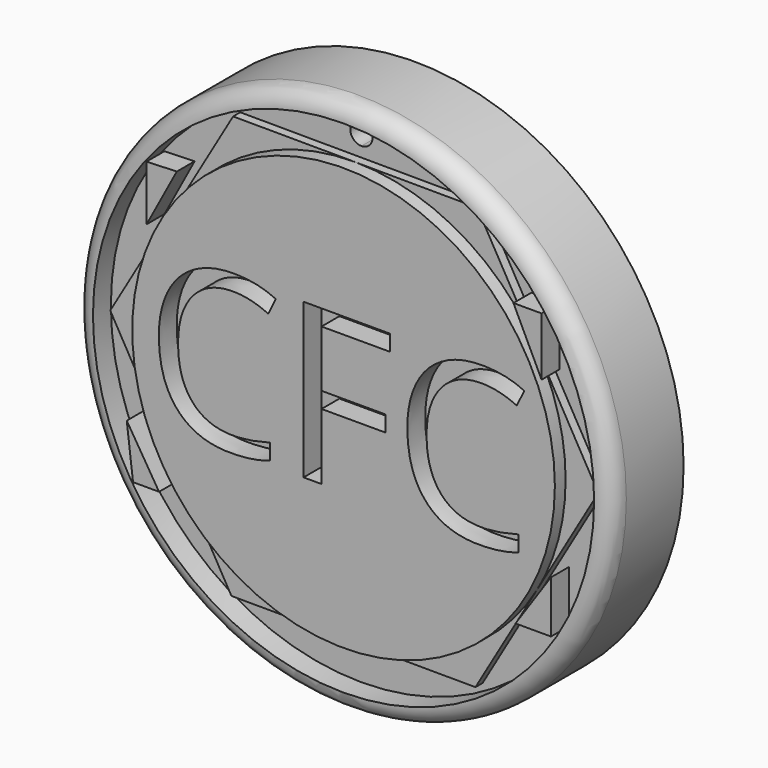
from build123d import *

# Parameters (mm, degrees)
F0_R          = 76.2
F1_DEPTH      = 25.4
F2_R          = 5.08
F3_DEPTH      = 6.35
F6_DEPTH      = 2.54
F7_R          = 59.9797814206
F8_DEPTH      = 3.81
F10_DEPTH     = 6.35
F11_TEXT_SIZE = 61.483415399
F12_DEPTH     = 6.35
F13_DEPTH     = 25.4


# Not quite as in the source:
# - Text() gives the source's letters only with a copy of the font that has no kerning and outlines rounded to 1/6400 em; it was checked with that copy


with BuildPart() as f1:
    # F0 (on Front) → F1 (new body)
    with BuildSketch(Plane.XZ):
        Circle(F0_R)
    extrude(amount=F1_DEPTH)

    # F2
    f2_edges = [f1.edges().sort_by_distance(p)[0] for p in [
        (-76.2, -25.4, 0),
    ]]
    fillet(f2_edges, radius=F2_R)

    # F3 (cut): a face of the model
    f3_faces = [f1.faces().sort_by_distance(p)[0] for p in [
        (0, -25.4, 0),
    ]]
    extrude(f3_faces, amount=-F3_DEPTH, mode=Mode.SUBTRACT)

    # F5 (on face) → F6 (join)
    with BuildSketch(Plane.XZ.offset(19.05)):
        Polygon((69.2581211383, -0.2796940148), (34.8712826912, 59.8394453168), (-34.3868384471, 60.1191393316), (-69.2581211383, 0.2796940148), (-34.8712826912, -59.8394453168), (34.3868384471, -60.1191393316), align=None)
    extrude(amount=F6_DEPTH)

    # F7 (on face) → F8 (join)
    with BuildSketch(Plane.XZ.offset(21.59)):
        Circle(F7_R)
    extrude(amount=F8_DEPTH)

    # F9 (on face) → F10 (join)
    with BuildSketch(Plane.XZ.offset(19.05)):
        Polygon((-47.3254956305, 43.6826720834), (-55.903814733, 43.3868691325), (-55.903814733, 27.7092475444), align=None)
        Polygon((-52.3541644216, -37.9592739046), (-61.5240931511, -23.169066757), (-59.7492679954, -37.9592739046), align=None)
        Polygon((56.2059618533, 41.9078469276), (48.2192486525, 41.9078469276), (56.2059618533, 25.3428146243), align=None)
        Polygon((58.8681958616, -23.169066757), (48.8108582795, -37.9592739046), (58.8681958616, -37.9592739046), align=None)
    extrude(amount=F10_DEPTH)

    # F11 (on face) → F12 (cut)
    with BuildSketch(Plane.XZ.offset(25.4)):
        with Locations((-56.1716337054, -21.0314466011)):
            Text('CFC', F11_TEXT_SIZE, font='Open Sans', text_align=(TextAlign.LEFT, TextAlign.BOTTOM))
    extrude(amount=-F12_DEPTH, mode=Mode.SUBTRACT)

    # F4 (on face) → F13 (cut)
    with BuildSketch(Plane.XZ.offset(19.05)):
        with BuildLine():
            ThreePointArc((0, 62.865), (2.2450640303, 63.7949359697), (3.175, 66.04))
            ThreePointArc((3.175, 66.04), (-2.2450640303, 68.2850640303), (0, 62.865))
        make_face()
    extrude(amount=-F13_DEPTH, mode=Mode.SUBTRACT)


solid = f1.part
